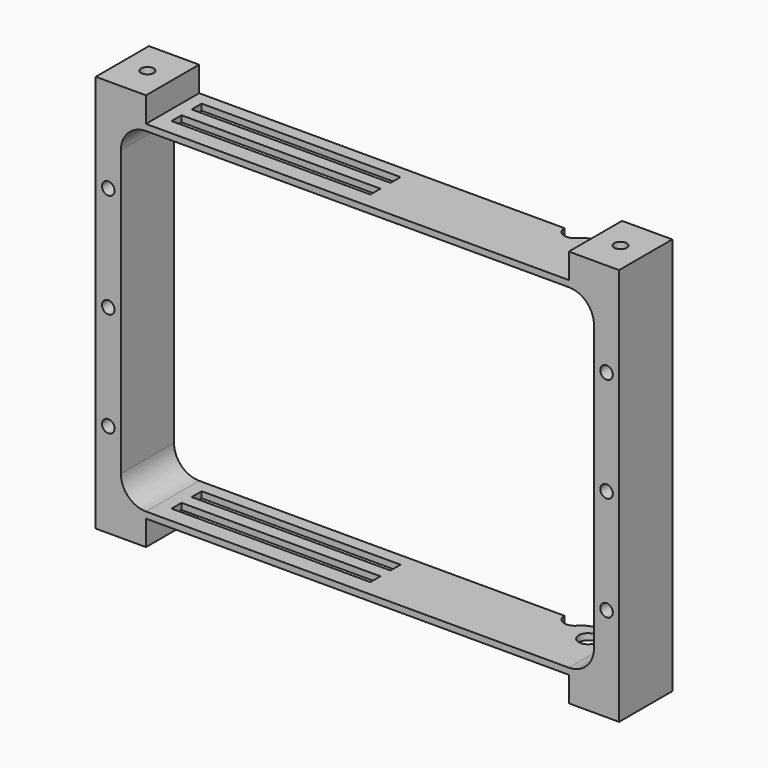
from build123d import *

# Parameters (mm, degrees)
F0_W      = 113
F0_H      = 80
F1_DEPTH  = 15.875
F2_R      = 6
F3_W      = 89
F3_H      = 3
F3_W_2    = 95
F3_R      = 1.5
F4_DEPTH  = 132
F5_R      = 1.5
F6_DEPTH  = 10
F7_W      = 42.9403819144
F7_H      = 7.4070980772
F8_DEPTH  = 1.5
F9_W      = 42.8083911538
F9_H      = 7.2430414148
F10_DEPTH = 1.5
F11_R     = 2.5
F12_DEPTH = 92
F13_R     = 2.25
F14_DEPTH = 200
F15_R     = 5
F16_R     = 1.5
F17_DEPTH = 9
F18_R     = 1.5
F19_DEPTH = 9
F20_R     = 1.5
F21_DEPTH = 9
F22_R     = 1.5
F23_DEPTH = 9


with BuildPart() as f1:
    # F0 (on Front) → F1 (new body)
    with BuildSketch(Plane.XZ):
        Polygon((-50.5, 47.5), (-62.5, 47.5), (-62.5, -47.5), (-50.5, -47.5), (-50.5, -41.5), (50.5, -41.5), (50.5, -47.5), (62.5, -47.5), (62.5, 47.5), (50.5, 47.5), (50.5, 41.5), (-50.5, 41.5), align=None)
        Rectangle(F0_W, F0_H, mode=Mode.SUBTRACT)
    extrude(amount=F1_DEPTH)

    # F2
    f2_edges = [f1.edges().sort_by_distance(p)[0] for p in [
        (56.5, -7.9375, 40),
        (56.5, -7.9375, -40),
        (-56.5, -7.9375, -40),
        (-56.5, -7.9375, 40),
    ]]
    fillet(f2_edges, radius=F2_R)

    # F3 (on face) → F4 (cut)
    with BuildSketch(Plane.XY.offset(41.5)):
        with Locations((-3, -4.5)):
            Rectangle(F3_W, F3_H)
        with Locations((0, -10.5)):
            Rectangle(F3_W_2, F3_H)
        with Locations((46, -4.5)):
            Circle(F3_R)
    extrude(amount=-F4_DEPTH, mode=Mode.SUBTRACT)

    # F5 (on face) → F6 (cut)
    with BuildSketch(Plane.XZ.offset(15.875)):
        with Locations((-59.5, 0)):
            Circle(F5_R)
        with Locations((59.5, 0)):
            Circle(F5_R)
        with Locations((59.5, -25)):
            Circle(F5_R)
        with Locations((59.5, 25)):
            Circle(F5_R)
        with Locations((-59.5, 25)):
            Circle(F5_R)
        with Locations((-59.5, -25)):
            Circle(F5_R)
    extrude(amount=-F6_DEPTH, mode=Mode.SUBTRACT)

    # F7 (on face) → F8 (join)
    with BuildSketch(Plane.XY.offset(41.5)):
        with Locations((21.4701909572, -3.7035490386)):
            Rectangle(F7_W, F7_H)
        Polygon((42.9403819144, -7.4070980772), (0, -7.4070980772), (0, -14.1382440925), (49.1435937583, -14.1382440925), (49.1435937583, -7.4070980772), align=None)
    extrude(amount=-F8_DEPTH)

    # F9 (on face) → F10 (join)
    with BuildSketch(Plane(origin=(0, 0, -41.5), x_dir=(1, 0, 0), z_dir=(0, 0, -1))):
        Polygon((49.0116067231, 15.875), (0, 15.875), (0, 7.2430414148), (42.8083911538, 7.2430414148), (49.0116067231, 7.2430414148), align=None)
        with Locations((21.4041955769, 3.6215207074)):
            Rectangle(F9_W, F9_H)
    extrude(amount=-F10_DEPTH)

    # F11 (on face) → F12 (cut)
    with BuildSketch(Plane.XY.offset(41.5)):
        with Locations((39.25, 0)):
            Circle(F11_R)
    extrude(amount=-F12_DEPTH, mode=Mode.SUBTRACT)

    # F13 (on face) → F14 (cut)
    with BuildSketch(Plane.XY.offset(41.5)):
        with Locations((46, -4.5)):
            Circle(F13_R)
    extrude(amount=-F14_DEPTH, mode=Mode.SUBTRACT)

    # F15
    f15_edges = [f1.edges().sort_by_distance(p)[0] for p in [
        (41.75, 0, 40.75),
        (41.75, 0, -40.75),
    ]]
    fillet(f15_edges, radius=F15_R)

    # F16 (on face) → F17 (cut)
    with BuildSketch(Plane.XY.offset(47.5)):
        with Locations((-56.5, -7.9375)):
            Circle(F16_R)
    extrude(amount=-F17_DEPTH, mode=Mode.SUBTRACT)

    # F18 (on face) → F19 (cut)
    with BuildSketch(Plane.XY.offset(47.5)):
        with Locations((56.5, -7.9375)):
            Circle(F18_R)
    extrude(amount=-F19_DEPTH, mode=Mode.SUBTRACT)

    # F20 (on face) → F21 (cut)
    with BuildSketch(Plane(origin=(0, 0, -47.5), x_dir=(1, 0, 0), z_dir=(0, 0, -1))):
        with Locations((-56.5, 7.9375)):
            Circle(F20_R)
    extrude(amount=-F21_DEPTH, mode=Mode.SUBTRACT)

    # F22 (on face) → F23 (cut)
    with BuildSketch(Plane(origin=(0, 0, -47.5), x_dir=(1, 0, 0), z_dir=(0, 0, -1))):
        with Locations((56.5, 7.9375)):
            Circle(F22_R)
    extrude(amount=-F23_DEPTH, mode=Mode.SUBTRACT)


solid = f1.part
